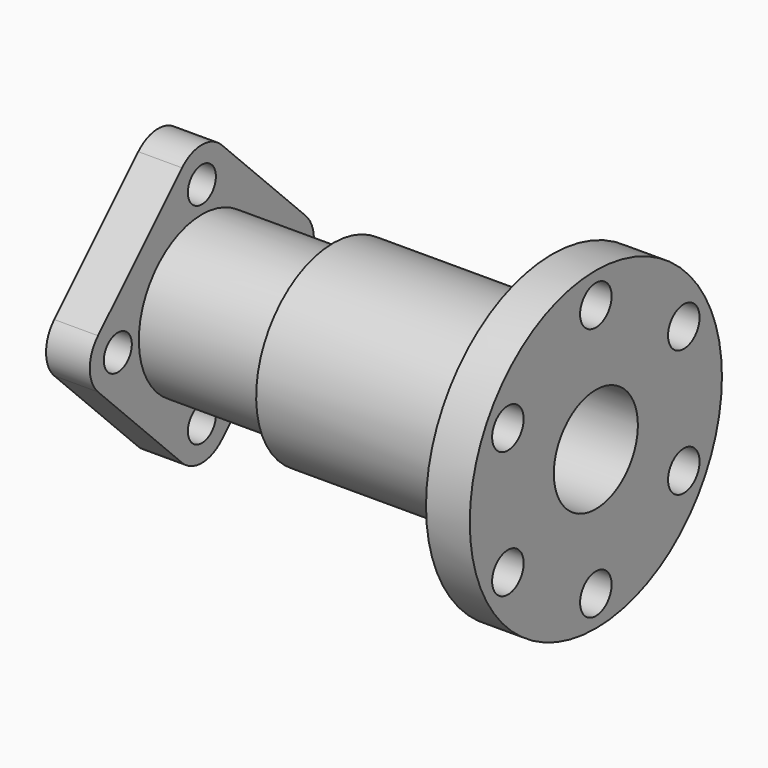
from build123d import *
from build123d import SkipClean  # not in build123d's __all__

# Parameters (mm, degrees)
F2_R     = 4.5
F3_DEPTH = 10.001
F4_R     = 4
F4_R_2   = 18
F4_R_3   = 8
F5_DEPTH = 10


with BuildPart() as f1:
    # F0 (on Front) → F1 (revolve)
    with BuildSketch(Plane.XZ):
        Polygon((-18.203094868, 18), (-18.203094868, 8), (21.796905132, 8), (21.796905132, 12), (71.796905132, 12), (71.796905132, 36), (61.796905132, 36), (61.796905132, 22), (11.796905132, 22), (11.796905132, 18), align=None)
    revolve(axis=Axis((24.6733184904, 0, 0), (1, 0, 0)))

    # F2 (on face) → F3 (cut, through all)
    with BuildSketch(Plane(origin=(61.796905132, 0, 0), x_dir=(0, -1, 0), z_dir=(-1, 0, 0))):
        with Locations((0, 29)):
            Circle(F2_R)
        with Locations((-25.1147367097, 14.5)):
            Circle(F2_R)
        with Locations((-25.1147367097, -14.5)):
            Circle(F2_R)
        with Locations((0, -29)):
            Circle(F2_R)
        with Locations((25.1147367097, -14.5)):
            Circle(F2_R)
        with Locations((25.1147367097, 14.5)):
            Circle(F2_R)
    extrude(amount=-F3_DEPTH, mode=Mode.SUBTRACT)

    # F4 (on face) → F5 (join)
    with BuildSketch(Plane(origin=(-18.203094868, 0, 0), x_dir=(0, -1, 0), z_dir=(-1, 0, 0))):
        with BuildLine():
            ThreePointArc((5.6568542495, 29.6568542495), (0, 32), (-5.6568542495, 29.6568542495))
            Line((-5.6568542495, 29.6568542495), (-29.6568542495, 5.6568542495))
            ThreePointArc((-29.6568542495, 5.6568542495), (-32, 0), (-29.6568542495, -5.6568542495))
            Line((-29.6568542495, -5.6568542495), (-5.6568542495, -29.6568542495))
            ThreePointArc((-5.6568542495, -29.6568542495), (0, -32), (5.6568542495, -29.6568542495))
            Line((5.6568542495, -29.6568542495), (29.6568542495, -5.6568542495))
            ThreePointArc((29.6568542495, -5.6568542495), (32, 0), (29.6568542495, 5.6568542495))
            Line((29.6568542495, 5.6568542495), (5.6568542495, 29.6568542495))
        make_face()
        with Locations((0, -24)):
            Circle(F4_R, mode=Mode.SUBTRACT)
        with Locations((-24, 0)):
            Circle(F4_R, mode=Mode.SUBTRACT)
        Circle(F4_R_2, mode=Mode.SUBTRACT)
        with Locations((24, 0)):
            Circle(F4_R, mode=Mode.SUBTRACT)
        with Locations((0, 24)):
            Circle(F4_R, mode=Mode.SUBTRACT)
        Circle(F4_R_2)
        Circle(F4_R_3, mode=Mode.SUBTRACT)
    with SkipClean():  # cleaning this boolean's faces spoils the solid; the shape is the same uncleaned
        extrude(amount=F5_DEPTH)


solid = f1.part
